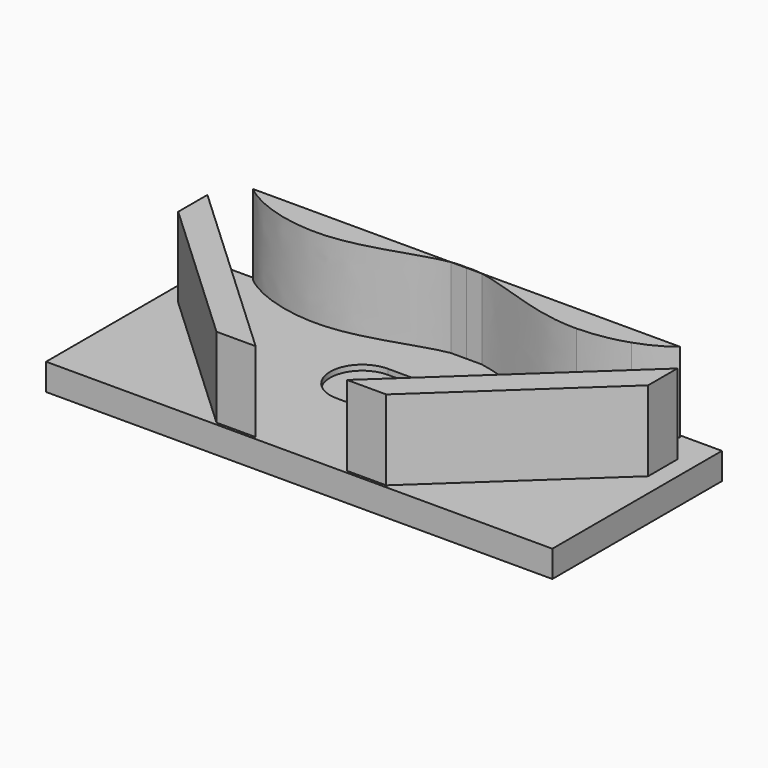
from build123d import *

# Parameters (mm, degrees)
F1_DEPTH         = 38.1
F2_E3_MIRRORCS_W = 109.4597315367
F2_E3_MIRRORCS_H = 38.1
F3_DEPTH         = 12.7
F2_E1_W          = 109.4624810587
F2_E1_H          = 38.1
F4_DEPTH         = 12.7
F6_DEPTH         = 38.1
F8_DEPTH         = 38.1
F9_W             = 241.0063309582
F9_H             = 100.9000240942
F10_DEPTH        = 12.7
F12_DEPTH        = 2.54
F14_DEPTH        = 38.1
F16_DEPTH        = 38.1


with BuildPart() as f1:
    # F0 (on Top) → F1 (new body)
    with BuildSketch(Plane.XY):
        with BuildLine():
            add(Edge.make_bspline(
                [(-7.3731541722, 88.9010522698), (-19.31236057, 87.050708456), (-56.3966234299, 68.9261750439), (-92.6223703207, 81.2413929209), (-101.6011297031, 88.9010522698)],
                knots=[0.1289921189, 0.1289921189, 0.1289921189, 0.1289921189, 0.4692924446, 0.7920589848, 0.7920589848, 0.7920589848, 0.7920589848], degree=3))
            Line((-7.3731541722, 88.9010522698), (-57.1511297031, 88.9010522698))
            Line((-57.1511297031, 88.9010522698), (-101.6011297031, 88.9010522698))
        make_face()
        with BuildLine():
            add(Edge.make_bspline(
                [(-0.0011297031, 88.9010522698), (-0.0010471723, 88.901093798), (-0.0009647066, 88.9011353269), (-0.0008823061, 88.9011768563)],
                knots=[0, 0, 0, 0, 1.61298e-05, 1.61298e-05, 1.61298e-05, 1.61298e-05], degree=3))
            Line((-0.0011297031, 88.9010522698), (-0.0006349067, 88.9010522698))
            add(Edge.make_bspline(
                [(-0.0006349067, 88.9010522747), (-0.0007174383, 88.9010938013), (-0.0007999048, 88.9011353285), (-0.0008823061, 88.9011768563)],
                knots=[0, 0, 0, 0, 1.61298e-05, 1.61298e-05, 1.61298e-05, 1.61298e-05], degree=3))
        make_face()
        with BuildLine():
            Line((-0.0038189409, 88.9010522698), (-0.0011297031, 88.9010522698))
            add(Edge.make_bspline(
                [(-0.0011297031, 88.9010522698), (-0.0010471723, 88.901093798), (-0.0009647066, 88.9011353269), (-0.0008823061, 88.9011768563)],
                knots=[0, 0, 0, 0, 1.61298e-05, 1.61298e-05, 1.61298e-05, 1.61298e-05], degree=3))
            add(Edge.make_bspline(
                [(-0.0008823061, 88.9011768563), (-0.0059560813, 88.9037338865), (-0.0107828824, 88.9062931167), (-0.0153641459, 88.9088540413)],
                knots=[1.61298e-05, 1.61298e-05, 1.61298e-05, 1.61298e-05, 0.0010093075, 0.0010093075, 0.0010093075, 0.0010093075], degree=3))
            add(Edge.make_bspline(
                [(-0.0038189409, 88.9010522698), (-0.0078539791, 88.9036552478), (-0.0117020651, 88.9062559427), (-0.0153641459, 88.9088540413)],
                knots=[0.0002095209, 0.0002095209, 0.0002095209, 0.0002095209, 0.001082787, 0.001082787, 0.001082787, 0.001082787], degree=3))
        make_face()
        with BuildLine():
            Line((-7.3731541722, 88.9010522698), (-0.0038189409, 88.9010522698))
            add(Edge.make_bspline(
                [(-0.0038189409, 88.9010522698), (-0.0078539791, 88.9036552478), (-0.0117020651, 88.9062559427), (-0.0153641459, 88.9088540413)],
                knots=[0.0002095209, 0.0002095209, 0.0002095209, 0.0002095209, 0.001082787, 0.001082787, 0.001082787, 0.001082787], degree=3))
            add(Edge.make_bspline(
                [(-0.0153641459, 88.9088540413), (-0.0906066198, 88.9509145567), (-0.0996162199, 88.9934321228), (-0.0487573192, 89.0341663757)],
                knots=[0.0010093075, 0.0010093075, 0.0010093075, 0.0010093075, 0.0173212144, 0.0173212144, 0.0173212144, 0.0173212144], degree=3))
            add(Edge.make_bspline(
                [(-0.0487573192, 89.0341663757), (-0.0385667228, 89.045259585), (-0.0248162276, 89.0561903305), (-0.0075963078, 89.0669286912)],
                knots=[0.0155197372, 0.0155197372, 0.0155197372, 0.0155197372, 0.0195117913, 0.0195117913, 0.0195117913, 0.0195117913], degree=3))
            add(Edge.make_bspline(
                [(-0.0075963078, 89.0669286912), (-0.5527500342, 89.3272580379), (-3.6107471198, 89.4841518814), (-7.3731541722, 88.9010522698)],
                knots=[0.0217531364, 0.0217531364, 0.0217531364, 0.0217531364, 0.1289921189, 0.1289921189, 0.1289921189, 0.1289921189], degree=3))
        make_face()
        with BuildLine():
            Line((7.358503656, 88.9011983473), (-0.0006349067, 88.9010522747))
            Line((-0.0006349067, 88.9010522698), (7.3594185793, 88.9010522698))
            add(Edge.make_bspline(
                [(7.358503656, 88.9011983473), (7.3588086257, 88.9011496596), (7.3591136001, 88.9011009671), (7.3594185793, 88.9010522698)],
                knots=[0.1288715075, 0.1288715075, 0.1288715075, 0.1288715075, 0.1288802405, 0.1288802405, 0.1288802405, 0.1288802405], degree=3))
        make_face()
        with BuildLine():
            add(Edge.make_bspline(
                [(-0.0006349067, 88.9010522747), (-0.0007174383, 88.9010938013), (-0.0007999048, 88.9011353285), (-0.0008823061, 88.9011768563)],
                knots=[0, 0, 0, 0, 1.61298e-05, 1.61298e-05, 1.61298e-05, 1.61298e-05], degree=3))
            Line((-0.0006349067, 88.9010522747), (7.358503656, 88.9011983473))
            add(Edge.make_bspline(
                [(6.9707545503, 88.9609054579), (7.0990916617, 88.9418687773), (7.2283658962, 88.9219745203), (7.358503656, 88.9011983473)],
                knots=[0.1251449345, 0.1251449345, 0.1251449345, 0.1251449345, 0.1288715075, 0.1288715075, 0.1288715075, 0.1288715075], degree=3))
            add(Edge.make_bspline(
                [(-0.0008839186, 89.0636547943), (0.5066620671, 89.3166069603), (3.3780640661, 89.4750941094), (6.9707545503, 88.9609054579)],
                knots=[0.0213043311, 0.0213043311, 0.0213043311, 0.0213043311, 0.1251592971, 0.1251592971, 0.1251592971, 0.1251592971], degree=3))
            add(Edge.make_bspline(
                [(-0.0008823061, 88.9011768563), (0.1078701091, 88.9559875108), (0.1031539373, 89.0118066991), (-0.0008839186, 89.0636547943)],
                knots=[1.61298e-05, 1.61298e-05, 1.61298e-05, 1.61298e-05, 0.0213043311, 0.0213043311, 0.0213043311, 0.0213043311], degree=3))
        make_face()
        with BuildLine():
            add(Edge.make_bspline(
                [(7.358503656, 88.9011983473), (7.3588086257, 88.9011496596), (7.3591136001, 88.9011009671), (7.3594185793, 88.9010522698)],
                knots=[0.1288715075, 0.1288715075, 0.1288715075, 0.1288715075, 0.1288802405, 0.1288802405, 0.1288802405, 0.1288802405], degree=3))
            Line((7.3594185793, 88.9010522698), (7.372333804, 88.9010522698))
            add(Edge.make_bspline(
                [(7.371389561, 88.901198603), (7.3717043037, 88.9011498305), (7.3720190514, 88.9011010527), (7.372333804, 88.9010522698)],
                knots=[0.1289921189, 0.1289921189, 0.1289921189, 0.1289921189, 0.1290010899, 0.1290010899, 0.1290010899, 0.1290010899], degree=3))
            Line((7.371389561, 88.901198603), (7.358503656, 88.9011983473))
        make_face()
        with BuildLine():
            Line((7.372333804, 88.9010522698), (7.3594185793, 88.9010522698))
            add(Edge.make_bspline(
                [(7.3594185793, 88.9010522698), (7.3633256696, 88.9004284077), (19.2537900005, 86.9997857358), (40.134248152, 76.8571245778), (60.7081186709, 76.2938170337), (62.4758923018, 76.3111989879)],
                knots=[0.1288802405, 0.1288802405, 0.1288802405, 0.1288802405, 0.1289921189, 0.4692924446, 0.5014907397, 0.5014907397, 0.5014907397, 0.5014907397], degree=3))
            add(Edge.make_bspline(
                [(7.372333804, 88.9010522698), (19.311636162, 87.0506013639), (40.1454385751, 76.8690456691), (60.7080947753, 76.2945495342), (62.4758923018, 76.3111989879)],
                knots=[0.1290010899, 0.1290010899, 0.1290010899, 0.1290010899, 0.4692924446, 0.5015061184, 0.5015061184, 0.5015061184, 0.5015061184], degree=3))
        make_face()
        with BuildLine():
            add(Edge.make_bspline(
                [(6.9707545503, 88.9609054579), (7.0990916617, 88.9418687773), (7.2283658962, 88.9219745203), (7.358503656, 88.9011983473)],
                knots=[0.1251449345, 0.1251449345, 0.1251449345, 0.1251449345, 0.1288715075, 0.1288715075, 0.1288715075, 0.1288715075], degree=3))
            Line((7.358503656, 88.9011983473), (7.371389561, 88.901198603))
            add(Edge.make_bspline(
                [(6.9707545503, 88.9609054579), (7.103344668, 88.9419290573), (7.2369171933, 88.9220364605), (7.371389561, 88.901198603)],
                knots=[0.1251592971, 0.1251592971, 0.1251592971, 0.1251592971, 0.1289921189, 0.1289921189, 0.1289921189, 0.1289921189], degree=3))
        make_face()
        with BuildLine():
            add(Edge.make_bspline(
                [(-0.0487573192, 89.0341663757), (-0.0363383579, 89.0441130537), (-0.0203496698, 89.0539533996), (-0.0008839186, 89.0636547943)],
                knots=[0.0173212144, 0.0173212144, 0.0173212144, 0.0173212144, 0.0213043311, 0.0213043311, 0.0213043311, 0.0213043311], degree=3))
            add(Edge.make_bspline(
                [(-0.0008839186, 89.0636547943), (-0.0030772808, 89.0647478738), (-0.0053147881, 89.0658391883), (-0.0075963078, 89.0669286912)],
                knots=[0.0213043311, 0.0213043311, 0.0213043311, 0.0213043311, 0.0217531364, 0.0217531364, 0.0217531364, 0.0217531364], degree=3))
            add(Edge.make_bspline(
                [(-0.0487573192, 89.0341663757), (-0.0385667228, 89.045259585), (-0.0248162276, 89.0561903305), (-0.0075963078, 89.0669286912)],
                knots=[0.0155197372, 0.0155197372, 0.0155197372, 0.0155197372, 0.0195117913, 0.0195117913, 0.0195117913, 0.0195117913], degree=3))
        make_face()
        with BuildLine():
            add(Edge.make_bspline(
                [(-0.0008839186, 89.0636547943), (-0.0030772808, 89.0647478738), (-0.0053147881, 89.0658391883), (-0.0075963078, 89.0669286912)],
                knots=[0.0213043311, 0.0213043311, 0.0213043311, 0.0213043311, 0.0217531364, 0.0217531364, 0.0217531364, 0.0217531364], degree=3))
            add(Edge.make_bspline(
                [(-0.0008839186, 89.0636547943), (0.5066620671, 89.3166069603), (3.3780640661, 89.4750941094), (6.9707545503, 88.9609054579)],
                knots=[0.0213043311, 0.0213043311, 0.0213043311, 0.0213043311, 0.1251592971, 0.1251592971, 0.1251592971, 0.1251592971], degree=3))
            add(Edge.make_bspline(
                [(-0.0075963078, 89.0669286912), (0.4480573981, 89.3510748377), (3.3329208845, 89.5005177095), (6.9707545503, 88.9609054579)],
                knots=[0.0195117913, 0.0195117913, 0.0195117913, 0.0195117913, 0.1251449345, 0.1251449345, 0.1251449345, 0.1251449345], degree=3))
        make_face()
        with BuildLine():
            add(Edge.make_bspline(
                [(7.371389561, 88.901198603), (7.3717043037, 88.9011498305), (7.3720190514, 88.9011010527), (7.372333804, 88.9010522698)],
                knots=[0.1289921189, 0.1289921189, 0.1289921189, 0.1289921189, 0.1290010899, 0.1290010899, 0.1290010899, 0.1290010899], degree=3))
            Line((7.372333804, 88.9010522698), (57.1488702969, 88.9010522698))
            Line((57.1488702969, 88.9010522698), (101.5970009453, 88.9010522698))
            add(Edge.make_bspline(
                [(101.5970009453, 88.9010522698), (101.5977890547, 88.9017244829), (101.5985770973, 88.9023967089), (101.5993650733, 88.9030689477)],
                knots=[0.7920306583, 0.7920306583, 0.7920306583, 0.7920306583, 0.7920589848, 0.7920589848, 0.7920589848, 0.7920589848], degree=3))
            Line((101.5993650733, 88.9030689477), (57.1493650821, 88.9021866532))
            Line((57.1493650821, 88.9021866532), (7.371389561, 88.901198603))
        make_face()
        with BuildLine():
            Line((57.1488702969, 88.9010522698), (7.372333804, 88.9010522698))
            add(Edge.make_bspline(
                [(7.372333804, 88.9010522698), (19.311636162, 87.0506013639), (40.1454385751, 76.8690456691), (60.7080947753, 76.2945495342), (62.4758923018, 76.3111989879)],
                knots=[0.1290010899, 0.1290010899, 0.1290010899, 0.1290010899, 0.4692924446, 0.5015061184, 0.5015061184, 0.5015061184, 0.5015061184], degree=3))
            add(Edge.make_bspline(
                [(62.4758923018, 76.3111989879), (70.6608896738, 76.3916794562), (78.6185391976, 77.8886425606), (85.5189213309, 80.2584115087)],
                knots=[0.5014907397, 0.5014907397, 0.5014907397, 0.5014907397, 0.6505725884, 0.6505725884, 0.6505725884, 0.6505725884], degree=3))
            add(Edge.make_bspline(
                [(85.5189213309, 80.2584115087), (92.0658589973, 82.5084423933), (97.6622116963, 85.5448972365), (101.5970009453, 88.9010522698)],
                knots=[0.650605221, 0.650605221, 0.650605221, 0.650605221, 0.7920306583, 0.7920306583, 0.7920306583, 0.7920306583], degree=3))
            Line((101.5970009453, 88.9010522698), (57.1488702969, 88.9010522698))
        make_face()
        with BuildLine():
            add(Edge.make_bspline(
                [(62.4758923018, 76.3111989879), (70.6608896738, 76.3916794562), (78.6185391976, 77.8886425606), (85.5189213309, 80.2584115087)],
                knots=[0.5014907397, 0.5014907397, 0.5014907397, 0.5014907397, 0.6505725884, 0.6505725884, 0.6505725884, 0.6505725884], degree=3))
            add(Edge.make_bspline(
                [(62.4758923018, 76.3111989879), (70.6580396422, 76.3882600096), (78.6167504823, 77.8862952047), (85.5189213309, 80.2584115087)],
                knots=[0.5015061184, 0.5015061184, 0.5015061184, 0.5015061184, 0.650605221, 0.650605221, 0.650605221, 0.650605221], degree=3))
        make_face()
    extrude(amount=F1_DEPTH)


with BuildPart() as f3:
    # F2_E3_MirrorCS (on explicit) → F3 (new body)
    with BuildSketch(Plane(origin=(31.75, 0, 0), x_dir=(0.7317397952, 0.6815840902, 0), z_dir=(0.6815840902, -0.7317397952, 0))):
        with Locations((54.7298657684, 19.05)):
            Rectangle(F2_E3_MIRRORCS_W, F2_E3_MIRRORCS_H)
    extrude(amount=F3_DEPTH)

    # F7 (on face) → F8 (join)
    with BuildSketch(Plane.XY.offset(38.1)):
        Polygon((40.406117946, -9.2930953996), (31.75, 0), (21.7730539089, -9.2930953996), align=None)
    extrude(amount=-F8_DEPTH)

    # F15 (on face) → F16 (cut)
    with BuildSketch(Plane.XY.offset(38.1)):
        Polygon((120.5021594878, 65.3129161372), (111.8460415418, 74.6060115367), (111.8460415418, 57.2501152433), align=None)
    extrude(amount=-F16_DEPTH, mode=Mode.SUBTRACT)


with BuildPart() as f4:
    # F2_E1 (on explicit) → F4 (new body)
    with BuildSketch(Plane(origin=(-31.75, 0, 0), x_dir=(-0.7317397957, 0.6815840897, 0), z_dir=(0.6815840897, 0.7317397957, 0))):
        with Locations((54.7312405293, 19.05)):
            Rectangle(F2_E1_W, F2_E1_H)
    extrude(amount=-F4_DEPTH)

    # F5 (on face) → F6 (join)
    with BuildSketch(Plane.XY.offset(38.1)):
        Polygon((-21.7730538874, -9.2930954059), (-31.75, 0), (-40.4061179392, -9.2930954059), align=None)
    extrude(amount=-F6_DEPTH)

    # F13 (on face) → F14 (cut)
    with BuildSketch(Plane.XY.offset(38.1)):
        Polygon((-111.8480535312, 57.2519892268), (-111.8480535312, 74.6078855084), (-120.5041714704, 65.3147901024), align=None)
    extrude(amount=-F14_DEPTH, mode=Mode.SUBTRACT)


with BuildPart() as f10:
    # F9 (on Top) → F10 (new body)
    with BuildSketch(Plane.XY):
        with Locations((-0.0010059913, 39.8869166412)):
            Rectangle(F9_W, F9_H)
    extrude(amount=-F10_DEPTH)

    # F11 (on face) → F12 (cut)
    with BuildSketch(Plane.XY):
        with BuildLine():
            Line((-17.7805990966, 33.8869045941), (-0.0004435264, 33.8869045941))
            Line((-0.0004435264, 33.8869045941), (-0.0008424617, 64.3669045941))
            Line((-0.0008424617, 64.3669045941), (-17.7805990966, 64.3669045941))
            ThreePointArc((-17.7805990966, 64.3669045941), (-33.0205990966, 49.1269045941), (-17.7805990966, 33.8869045941))
        make_face()
        with BuildLine():
            Line((-0.0008424617, 64.3669045941), (-0.0004435264, 33.8869045941))
            Line((-0.0004435264, 33.8869045941), (17.7794009034, 33.8869045941))
            ThreePointArc((17.7794009034, 33.8869045941), (33.0194009034, 49.1269045941), (17.7794009034, 64.3669045941))
            Line((17.7794009034, 64.3669045941), (-0.0008424617, 64.3669045941))
        make_face()
    extrude(amount=-F12_DEPTH, mode=Mode.SUBTRACT)


solid = Compound([f1.part, f3.part, f4.part, f10.part])
